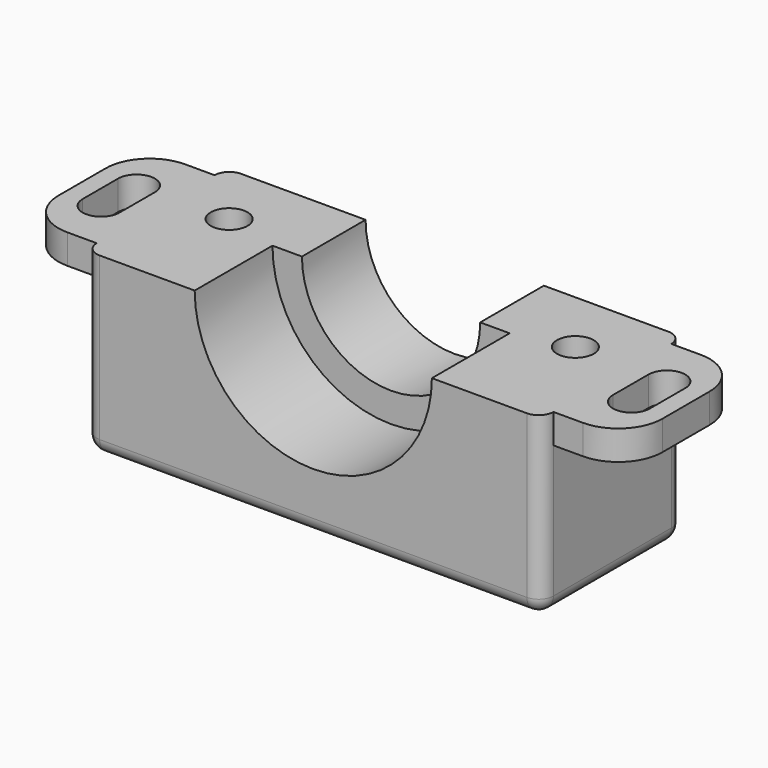
from build123d import *

# Parameters (mm, degrees)
F0_W      = 25
F0_H      = 12
F1_DEPTH  = 12
F2_R      = 8.05
F3_DEPTH  = 6.6
F4_R      = 6.05
F5_DEPTH  = 5.4
F6_W      = 12
F6_H      = 12
F7_DEPTH  = 3
F8_W      = 12
F8_H      = 12
F9_DEPTH  = 3
F10_R     = 1.25
F11_DEPTH = 25
F12_SIZE  = 1.5
F13_R     = 0.99999
F14_W     = 10
F14_H     = 2
F15_DEPTH = 5
F16_W     = 10
F16_H     = 2
F17_DEPTH = 5
F19_DEPTH = 2
F20_R     = 3


# Not quite as in the source:
# - a fillet or chamfer is up to 0.001 mm smaller than in the source, because OpenCascade refuses the exact size


with BuildPart() as f1:
    # F0 (on Top) → F1 (new body)
    with BuildSketch(Plane.XY):
        with Locations((12.5, 6)):
            Rectangle(F0_W, F0_H)
    extrude(amount=F1_DEPTH)

    # F2 (on face) → F3 (cut)
    with BuildSketch(Plane.XZ):
        with Locations((12.5, 12)):
            Circle(F2_R)
    extrude(amount=-F3_DEPTH, mode=Mode.SUBTRACT)

    # F4 (on face) → F5 (cut)
    with BuildSketch(Plane(origin=(0, 12, 0), x_dir=(-1, 0, 0), z_dir=(0, 1, 0))):
        with Locations((-12.5, 12)):
            Circle(F4_R)
    extrude(amount=-F5_DEPTH, mode=Mode.SUBTRACT)

    # F6 (on face) → F7 (join)
    with BuildSketch(Plane(origin=(0, 0, 0), x_dir=(0, -1, 0), z_dir=(-1, 0, 0))):
        with Locations((-6, 6)):
            Rectangle(F6_W, F6_H)
    extrude(amount=F7_DEPTH)

    # F8 (on face) → F9 (join)
    with BuildSketch(Plane.YZ.offset(25)):
        with Locations((6, 6)):
            Rectangle(F8_W, F8_H)
    extrude(amount=F9_DEPTH)

    # F10 (on face) → F11 (cut)
    with BuildSketch(Plane.XY.offset(12)):
        with Locations((0.75, 7.55)):
            Circle(F10_R)
        with Locations((24.25, 7.55)):
            Circle(F10_R)
    extrude(amount=-F11_DEPTH, mode=Mode.SUBTRACT)

    # F12
    f12_edges = [f1.edges().sort_by_distance(p)[0] for p in [
        (23, 7.55, 0),
        (-0.5, 7.55, 0),
    ]]
    chamfer(f12_edges, length=F12_SIZE)

    # F13 (radius 1 in the source; OpenCascade refuses exactly that, so slightly less here)
    f13_edges = [f1.edges().sort_by_distance(p)[0] for p in [
        (28, 6, 0),
        (-3, 6, 0),
        (28, 12, 6),
        (12.5, 12, 0),
        (-3, 12, 6),
        (-3, 0, 6),
        (12.5, 0, 0),
        (28, 0, 6),
    ]]
    fillet(f13_edges, radius=F13_R)

    # F14 (on face) → F15 (join)
    with BuildSketch(Plane.YZ.offset(28)):
        with Locations((6, 11)):
            Rectangle(F14_W, F14_H)
    extrude(amount=F15_DEPTH)

    # F16 (on face) → F17 (join)
    with BuildSketch(Plane(origin=(-3, 0, 0), x_dir=(0, -1, 0), z_dir=(-1, 0, 0))):
        with Locations((-6, 11)):
            Rectangle(F16_W, F16_H)
    extrude(amount=F17_DEPTH)

    # F18 (on face) → F19 (cut, through all)
    with BuildSketch(Plane.XY.offset(12)):
        with BuildLine():
            ThreePointArc((-4.25, 7.5), (-5.5, 8.75), (-6.75, 7.5))
            Line((-6.75, 7.5), (-6.75, 4.5))
            ThreePointArc((-6.75, 4.5), (-5.5, 3.25), (-4.25, 4.5))
            Line((-4.25, 4.5), (-4.25, 7.5))
        make_face()
        with BuildLine():
            ThreePointArc((31.75, 7.5), (30.5, 8.75), (29.25, 7.5))
            Line((29.25, 7.5), (29.25, 4.5))
            ThreePointArc((29.25, 4.5), (30.5, 3.25), (31.75, 4.5))
            Line((31.75, 4.5), (31.75, 7.5))
        make_face()
    extrude(amount=-F19_DEPTH, mode=Mode.SUBTRACT)

    # F20
    f20_edges = [f1.edges().sort_by_distance(p)[0] for p in [
        (-8, 11, 11),
        (-8, 1, 11),
        (33, 11, 11),
        (33, 1, 11),
    ]]
    fillet(f20_edges, radius=F20_R)


solid = f1.part
